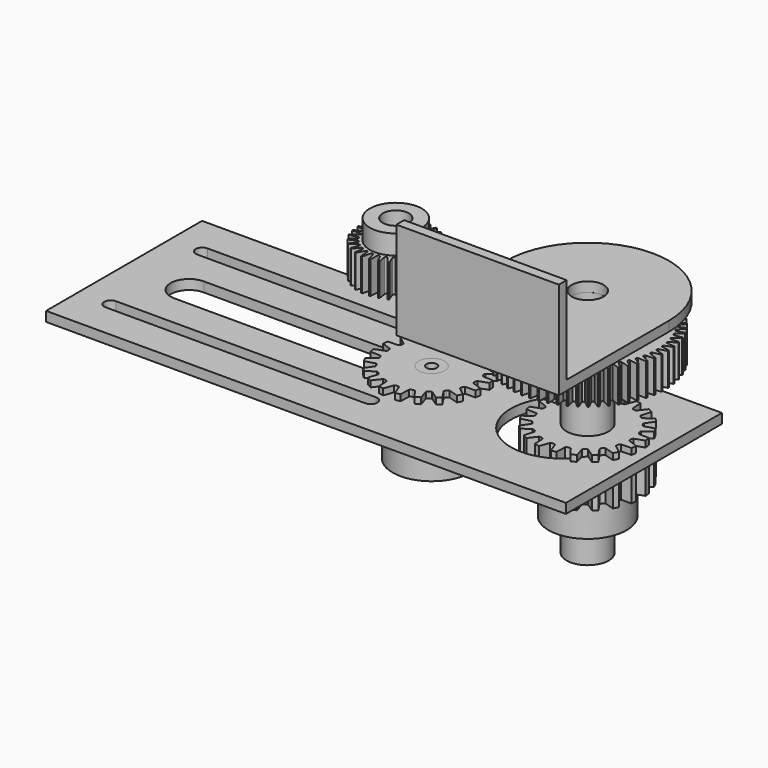
from build123d import *

# Parameters (mm, degrees)
F7_DEPTH         = 10
F7_COPIES_COUNT  = 60
F0_W             = 1.5
F0_H             = 9
F12_DEPTH        = 15
F12_COPIES_COUNT = 20
F13_DEPTH        = 15
F13_COPIES_COUNT = 20
F0_W_2           = 2.4
F0_H_2           = 25
F16_DEPTH        = 10
F16_COPIES_COUNT = 30
F1_W             = 160
F1_H             = 60
F1_R             = 16
F17_DEPTH        = 3
F18_R            = 4.9
F19_DEPTH        = 30
F20_T            = -3


# Not quite as in the source:
# - a pattern or mirror of a feature is missing from the dataset's text; its kind, count and spacing are read off the source's solid


with BuildPart() as f2:
    # F0 (on Front) → F2 (revolve)
    with BuildSketch(Plane.XZ):
        Polygon((-81.019856, -30.1045326953), (-81.019856, -21.1045326953), (-81.019856, 37.8954673047), (-82.619856, 37.8954673047), (-82.619856, 31.8954673047), (-82.619856, 21.8954673047), (-82.619856, 4.8954673047), (-82.619856, -20.1045326953), (-82.619856, -30.1045326953), align=None)
    revolve(axis=Axis((-76.119856, 0, 8.3954673047), (0, 0, -1)))


with BuildPart() as f3:
    # F0 (on Front) → F3 (revolve)
    with BuildSketch(Plane.XZ):
        Polygon((-136.119856, -20.1045326953), (-128.119856, -20.1045326953), (-128.119856, 4.8954673047), (-140.619856, 4.8954673047), (-140.619856, -10.1045326953), (-136.119856, -10.1045326953), align=None)
    revolve(axis=Axis((-124.119856, 0, -7.6045326953), (0, 0, -1)))

    # F9 (on face) → F13 (cut, through all)
    with BuildSketch(Plane(origin=(0, 0, -10.1045326953), x_dir=(1, 0, 0), z_dir=(0, 0, -1))):
        with BuildLine():
            Line((-124.119856, -16.5), (-124.119856, -13.2379025166))
            ThreePointArc((-124.119856, -13.2379025166), (-124.5137787785, -13.2996987755), (-124.869856, -13.4791505667))
            Line((-124.869856, -13.4791505667), (-125.93298663, -16.4000779668))
            ThreePointArc((-125.93298663, -16.4000779668), (-125.0277969527, -16.4750005532), (-124.119856, -16.5))
        make_face()
        with BuildLine():
            ThreePointArc((-123.369856, -13.4791505667), (-123.7259332215, -13.2996987755), (-124.119856, -13.2379025166))
            Line((-124.119856, -13.2379025166), (-124.119856, -16.5))
            ThreePointArc((-124.119856, -16.5), (-123.2119150473, -16.4750005532), (-122.3067253698, -16.4000779668))
            Line((-122.3067253698, -16.4000779668), (-123.369856, -13.4791505667))
        make_face()
    f13 = extrude(amount=-F13_DEPTH, mode=Mode.SUBTRACT)

    # F13_copies: F13 ×20 about axis
    f13_copies_axis = Axis((-124.119856, 0, 0), (0, 0, 1))
    for i in range(1, F13_COPIES_COUNT):
        add(f13.rotate(f13_copies_axis, i * 360 / F13_COPIES_COUNT), mode=Mode.SUBTRACT)


with BuildPart() as f4:
    # F0 (on Front) → F4 (revolve)
    with BuildSketch(Plane.XZ):
        Polygon((-88.119856, -20.1045326953), (-82.619856, -20.1045326953), (-82.619856, 4.8954673047), (-92.619856, 4.8954673047), (-92.619856, -10.1045326953), (-88.119856, -10.1045326953), align=None)
    revolve(axis=Axis((-76.119856, 0, 8.3954673047), (0, 0, -1)))

    # F8 (on face) → F12 (cut, through all)
    with BuildSketch(Plane(origin=(0, 0, -10.1045326953), x_dir=(1, 0, 0), z_dir=(0, 0, -1))):
        with BuildLine():
            ThreePointArc((-59.7197780331, -1.8131306301), (-59.6263627283, 0), (-59.7197780331, 1.8131306301))
            Line((-59.7197780331, 1.8131306301), (-62.6407054332, 0.75))
            Line((-62.6407054332, 0.75), (-62.6407054332, -0.75))
            Line((-62.6407054332, -0.75), (-59.7197780331, -1.8131306301))
        make_face()
        with BuildLine():
            Line((-62.6407054332, -0.75), (-62.6407054332, 0.75))
            ThreePointArc((-62.6407054332, 0.75), (-62.8984510343, 0), (-62.6407054332, -0.75))
        make_face()
        with BuildLine():
            ThreePointArc((-59.619856, 0), (-59.6448554468, 0.9079409527), (-59.7197780332, 1.8131306301))
            ThreePointArc((-59.7197780331, 1.8131306301), (-59.6263627283, 0), (-59.7197780331, -1.8131306301))
            ThreePointArc((-59.7197780332, -1.8131306301), (-59.6448554468, -0.9079409527), (-59.619856, 0))
        make_face()
    f12 = extrude(amount=-F12_DEPTH, mode=Mode.SUBTRACT)

    # F12_copies: F12 ×20 about axis
    f12_copies_axis = Axis((-76.119856, 0, 0), (0, 0, 1))
    for i in range(1, F12_COPIES_COUNT):
        add(f12.rotate(f12_copies_axis, i * 360 / F12_COPIES_COUNT), mode=Mode.SUBTRACT)


with BuildPart() as f5:
    # F0 (on Front) → F5 (revolve)
    with BuildSketch(Plane.XZ):
        Polygon((-82.619856, 31.8954673047), (-82.619856, 37.8954673047), (-93.619856, 37.8954673047), (-93.619856, 31.8954673047), (-100.044856, 31.8954673047), (-100.044856, 21.8954673047), (-82.619856, 21.8954673047), align=None)
    revolve(axis=Axis((-76.119856, 0, 8.3954673047), (0, 0, -1)))

    # F6 (on face) → F7 (cut, through all)
    with BuildSketch(Plane.XY.offset(31.8954673047)):
        with BuildLine():
            ThreePointArc((-77.1595523631, -23.9023985506), (-76.1198559999, -23.925), (-75.0801596368, -23.9023985506))
            Line((-75.0801596368, -23.9023985506), (-75.744856, -21.4217179516))
            ThreePointArc((-75.744856, -21.4217179516), (-76.119856, -21.3057444347), (-76.494856, -21.4217179516))
            Line((-76.494856, -21.4217179516), (-77.1595523631, -23.9023985506))
        make_face()
    f7 = extrude(amount=-F7_DEPTH, mode=Mode.SUBTRACT)

    # F7_copies: F7 ×60 about axis
    f7_copies_axis = Axis((-76.119856, 0, 0), (0, 0, 1))
    for i in range(1, F7_COPIES_COUNT):
        add(f7.rotate(f7_copies_axis, i * 360 / F7_COPIES_COUNT), mode=Mode.SUBTRACT)


with BuildPart() as f10:
    # F0 (on Front) → F10 (revolve)
    with BuildSketch(Plane.XZ):
        Polygon((-146.8324561119, 25.3721504574), (-139.1698714831, 25.3721504574), (-139.1698714831, 41.3721504574), (-143.1574561119, 41.3721504574), (-143.1574561119, 35.3721504574), (-146.8324561119, 35.3721504574), align=None)
    revolve(axis=Axis((-135.1574561119, 0, 33.3721504574), (0, 0, -1)))

    # F15 (on face) → F16 (cut, through all)
    with BuildSketch(Plane.XY.offset(35.3721504574)):
        with BuildLine():
            ThreePointArc((-136.1920755323, -11.6290664997), (-135.1574561119, -11.675), (-134.1228366915, -11.6290664997))
            Line((-134.1228366915, -11.6290664997), (-134.7824561119, -9.1673333091))
            ThreePointArc((-134.7824561119, -9.1673333091), (-135.1574561119, -8.912317278), (-135.5324561119, -9.1673333091))
            Line((-135.5324561119, -9.1673333091), (-136.1920755323, -11.6290664997))
        make_face()
    f16 = extrude(amount=-F16_DEPTH, mode=Mode.SUBTRACT)

    # F16_copies: F16 ×30 about axis
    f16_copies_axis = Axis((-135.157456, 0, 0), (0, 0, 1))
    for i in range(1, F16_COPIES_COUNT):
        add(f16.rotate(f16_copies_axis, i * 360 / F16_COPIES_COUNT), mode=Mode.SUBTRACT)


with BuildPart() as f11:
    # F0 (on Front) → F11 (revolve)
    with BuildSketch(Plane.XZ):
        with Locations((-80.269856, -25.6045326953)):
            Rectangle(F0_W, F0_H)
    revolve(axis=Axis((-76.119856, 0, 8.3954673047), (0, 0, -1)))


with BuildPart() as f14:
    # F0 (on Front) → F14 (revolve)
    with BuildSketch(Plane.XZ):
        with Locations((-126.919856, -7.6045326953)):
            Rectangle(F0_W_2, F0_H_2)
    revolve(axis=Axis((-124.119856, 0, -7.6045326953), (0, 0, -1)))


with BuildPart() as f17:
    # F1 (on Top) → F17 (new body)
    with BuildSketch(Plane.XY):
        with Locations((-136.6810971498, -2.6440789869)):
            Rectangle(F1_W, F1_H)
        with BuildLine():
            ThreePointArc((-126.6810971498, -18.2190789869), (-124.6560971498, -20.2440789869), (-126.6810971498, -22.2690789869))
            Line((-126.6810971498, -22.2690789869), (-206.6810971498, -22.2690789869))
            ThreePointArc((-206.6810971498, -22.2690789869), (-208.7060971498, -20.2440789869), (-206.6810971498, -18.2190789869))
            Line((-206.6810971498, -18.2190789869), (-126.6810971498, -18.2190789869))
        make_face(mode=Mode.SUBTRACT)
        with BuildLine():
            Line((-136.6810971498, -8.3091505284), (-196.6810971498, -8.3091505284))
            ThreePointArc((-196.6810971498, -8.3091505284), (-202.3461686913, -2.6440789869), (-196.6810971498, 3.0209925545))
            Line((-196.6810971498, 3.0209925545), (-136.6810971498, 3.0209925545))
            ThreePointArc((-136.6810971498, 3.0209925545), (-131.0160256084, -2.6440789869), (-136.6810971498, -8.3091505284))
        make_face(mode=Mode.SUBTRACT)
        with BuildLine():
            ThreePointArc((-206.6810971498, 12.9309210131), (-208.7060971498, 14.9559210131), (-206.6810971498, 16.9809210131))
            Line((-206.6810971498, 16.9809210131), (-126.6810971498, 16.9809210131))
            ThreePointArc((-126.6810971498, 16.9809210131), (-124.6560971498, 14.9559210131), (-126.6810971498, 12.9309210131))
            Line((-126.6810971498, 12.9309210131), (-206.6810971498, 12.9309210131))
        make_face(mode=Mode.SUBTRACT)
        with Locations((-81.6810971498, -2.6440789869)):
            Circle(F1_R, mode=Mode.SUBTRACT)
    extrude(amount=F17_DEPTH)


with BuildPart() as f19:
    # F18 (on face) → F19 (new body)
    with BuildSketch(Plane.XY.offset(37.8954673047)):
        with BuildLine():
            Line((-101.119856, -42.35611), (-51.119856, -42.35611))
            Line((-51.119856, -42.35611), (-51.119856, 0))
            ThreePointArc((-51.119856, 0), (-76.119856, 25), (-101.119856, 0))
            Line((-101.119856, 0), (-101.119856, -42.35611))
        make_face()
        with Locations((-76.119856, 0)):
            Circle(F18_R, mode=Mode.SUBTRACT)
    extrude(amount=F19_DEPTH)

    # F20
    f20_openings = [f19.faces().sort_by_distance(p)[0] for p in [
        (-76.119856, 25, 52.895467),
        (-81.019856, 0, 52.895467),
        (-76.119856, -11.38655, 67.895467),
        (-51.119856, -21.178055, 52.895467),
        (-101.119856, -21.178055, 52.895467),
    ]]
    offset(amount=F20_T, openings=f20_openings)


solid = Compound([f2.part, f3.part, f4.part, f5.part, f10.part, f11.part, f14.part, f17.part, f19.part])
